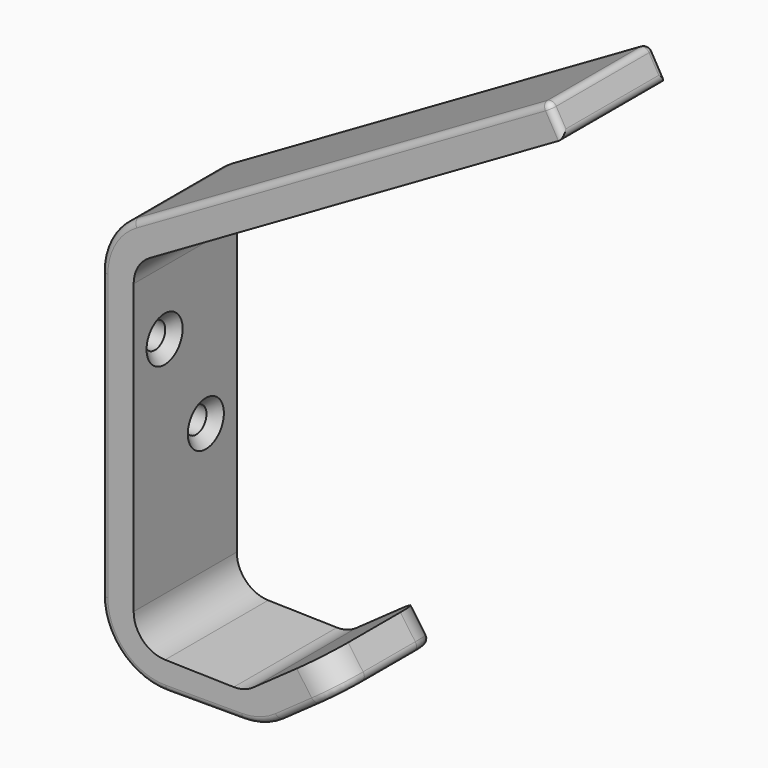
from build123d import *

# Parameters (mm, degrees)
F1_DEPTH       = 20
F2_R           = 10
F3_R           = 10
F4_R           = 5
F5_R           = 5
F6_R           = 5
F8_D           = 4
F8_DEPTH       = 12
F8_CSINK_D     = 7
F8_CSINK_ANGLE = 90
F8_TIP         = 1.2017212381
F9_T1_DEPTH    = 30.0048285071
F10_R          = 1
F11_T1_DEPTH   = 25
F11_T3_DEPTH   = 18
F11_T5_DEPTH   = 6.5
F11_T8_ANGLE   = 90
F11_T10_ANGLE  = 90


# Not quite as in the source:
# - a fillet or chamfer that OpenCascade refuses, or shapes differently, is made with other operations: its cross-section is extruded or revolved along the edge and cut away or added


with BuildPart() as f1:
    # F0 (on Front) → F1 (new body)
    with BuildSketch(Plane.XZ):
        Polygon((13.3003787555, -46.1032405242), (38.3003787555, -46.1032405242), (50.5316518247, -37.4287553132), (47.6391971652, -33.3503112419), (35.4933471628, -41.9642139506), (18.3003787555, -41.5471586402), (18.3003787555, 11.0100081298), (85.0824110582, 49.5666324568), (82.5824110582, 53.8967594758), (13.3003787555, 13.8967594758), align=None)
    extrude(amount=F1_DEPTH)

    # F2
    f2_edges = [f1.edges().sort_by_distance(p)[0] for p in [
        (13.300379, -10, 13.896759),
        (13.300379, -10, -46.103241),
    ]]
    fillet(f2_edges, radius=F2_R)

    # F3
    f3_edges = [f1.edges().sort_by_distance(p)[0] for p in [
        (38.300379, -10, -46.103241),
    ]]
    fillet(f3_edges, radius=F3_R)

    # F4
    f4_edges = [f1.edges().sort_by_distance(p)[0] for p in [
        (18.300379, -10, 11.010008),
    ]]
    fillet(f4_edges, radius=F4_R)

    # F5
    f5_edges = [f1.edges().sort_by_distance(p)[0] for p in [
        (18.300379, -10, -41.547159),
    ]]
    fillet(f5_edges, radius=F5_R)

    # F6
    f6_edges = [f1.edges().sort_by_distance(p)[0] for p in [
        (35.493347, -10, -41.964214),
    ]]
    fillet(f6_edges, radius=F6_R)

    # F8
    with Locations(Plane.YZ.offset(18.3003787555)):
        with Locations((-6, -16.6669744052), (-14, -1.8767432161)):
            CounterSinkHole(F8_D / 2, F8_CSINK_D / 2, depth=F8_DEPTH, counter_sink_angle=F8_CSINK_ANGLE)
            with Locations((0, 0, -(F8_DEPTH + F8_TIP / 2))):  # 118° drill point
                Cone(0, F8_D / 2, F8_TIP, mode=Mode.SUBTRACT)

    # F9: fillet of radius 5 on 2 edges, made by hand

    # F9_s2 → F9_t1 (cut)
    with BuildSketch(Plane(origin=(41.804493112, 0, -58.9455349028), x_dir=(0, 1, 0), z_dir=(-0.5784909319, 0, 0.8156888143))):
        with BuildLine():
            ThreePointArc((0.0004, -14.5649419331), (-1.4644660941, -18.1014415245), (-5.0009656854, -19.5663076185))
            Line((-5.0009656854, -19.5663076185), (-5.0009656854, -20.0664441871))
            ThreePointArc((-5.0009656854, -20.0664441871), (-2.5004828427, -20.0660441871), (0, -20.0660441871))
            Line((0, -20.0660441871), (0.5001365685, -19.5659076185))
            ThreePointArc((0.5001365685, -19.5659076185), (0.5001365685, -17.0654247758), (0.5005365685, -14.5649419331))
            Line((0.5005365685, -14.5649419331), (0.0004, -14.5649419331))
        make_face()
        with BuildLine():
            ThreePointArc((-14.9990343146, -19.5663076185), (-18.5355339059, -18.1014415245), (-20.0004, -14.5649419331))
            Line((-20.0004, -14.5649419331), (-20.5005365685, -14.5649419331))
            ThreePointArc((-20.5005365685, -14.5649419331), (-20.5001365685, -17.0654247758), (-20.5001365685, -19.5659076185))
            Line((-20.5001365685, -19.5659076185), (-20, -20.0660441871))
            ThreePointArc((-20, -20.0660441871), (-17.4995171573, -20.0660441871), (-14.9990343146, -20.0664441871))
            Line((-14.9990343146, -20.0664441871), (-14.9990343146, -19.5663076185))
        make_face()
    extrude(amount=F9_T1_DEPTH, mode=Mode.SUBTRACT)

    # F10
    f10_edges = [f1.edges().sort_by_distance(p)[0] for p in [
        (50.441395, -20, 35.340135),
        (14.640125, -20, 13.123257),
        (13.300379, -20, -13.989992),
        (16.229311, -20, -43.174308),
        (29.207344, -20, -46.103241),
        (38.150024, -20, -45.631327),
        (43.701617, -20, -42.272653),
    ]]
    fillet(f10_edges, radius=F10_R)

    # F11: fillet of radius 1 on 6 edges, made by hand

    # F11_s2 → F11_t1 (cut)
    with BuildSketch(Plane.XZ.offset(-2.5)):
        with BuildLine():
            ThreePointArc((84.2163856545, 49.0666324568), (84.6823114807, 49.6738388155), (84.5824110582, 50.4326578606))
            Line((84.5824110582, 50.4326578606), (85.0824110582, 49.5666324568))
            Line((85.0824110582, 49.5666324568), (84.2163856545, 49.0666324568))
        make_face()
    extrude(amount=F11_T1_DEPTH, mode=Mode.SUBTRACT)

    # F11_s4 → F11_t3 (cut)
    with BuildSketch(Plane.XZ.offset(1)):
        with BuildLine():
            ThreePointArc((83.0824110582, 53.030734072), (82.4752046996, 53.4966598983), (81.7163856545, 53.3967594758))
            Line((81.7163856545, 53.3967594758), (82.5824110582, 53.8967594758))
            Line((82.5824110582, 53.8967594758), (83.0824110582, 53.030734072))
        make_face()
    extrude(amount=F11_T3_DEPTH, mode=Mode.SUBTRACT)

    # F11_s6 → F11_t5 (cut)
    with BuildSketch(Plane(origin=(1.0576213207, 0, -1.8318538627), x_dir=(0, 1, 0), z_dir=(-0.5, 0, 0.8660254038))):
        with BuildLine():
            ThreePointArc((0, -97.4668456201), (-0.2928932188, -98.1739524013), (-1, -98.4668456201))
            Line((-1, -98.4668456201), (0, -98.4668456201))
            Line((0, -98.4668456201), (0, -97.4668456201))
        make_face()
        with BuildLine():
            ThreePointArc((-19, -98.4668456201), (-19.7071067812, -98.1739524013), (-20, -97.4668456201))
            Line((-20, -97.4668456201), (-20, -98.4668456201))
            Line((-20, -98.4668456201), (-19, -98.4668456201))
        make_face()
    extrude(amount=F11_T5_DEPTH, mode=Mode.SUBTRACT)

    # F11_s7 → F11_t8 (revolve, cut)
    with BuildSketch(Plane.XZ.offset(1)):
        with BuildLine():
            ThreePointArc((81.7163856545, 53.3967594758), (82.4752046996, 53.4966598983), (83.0824110582, 53.030734072))
            Line((83.0824110582, 53.030734072), (82.5824110582, 53.8967594758))
            Line((82.5824110582, 53.8967594758), (81.7163856545, 53.3967594758))
        make_face()
    revolve(axis=Axis((83.0824110582, -1, 53.030734072), (-0.8660254038, 0, -0.5)), revolution_arc=F11_T8_ANGLE, mode=Mode.SUBTRACT)

    # F11_s9 → F11_t10 (revolve, cut)
    with BuildSketch(Plane.XZ.offset(19)):
        with BuildLine():
            ThreePointArc((83.0824110582, 53.030734072), (82.4752046996, 53.4966598983), (81.7163856545, 53.3967594758))
            Line((81.7163856545, 53.3967594758), (82.5824110582, 53.8967594758))
            Line((82.5824110582, 53.8967594758), (83.0824110582, 53.030734072))
        make_face()
    revolve(axis=Axis((83.0824110582, -19, 53.030734072), (0.8660254038, 0, 0.5)), revolution_arc=F11_T10_ANGLE, mode=Mode.SUBTRACT)


solid = f1.part
